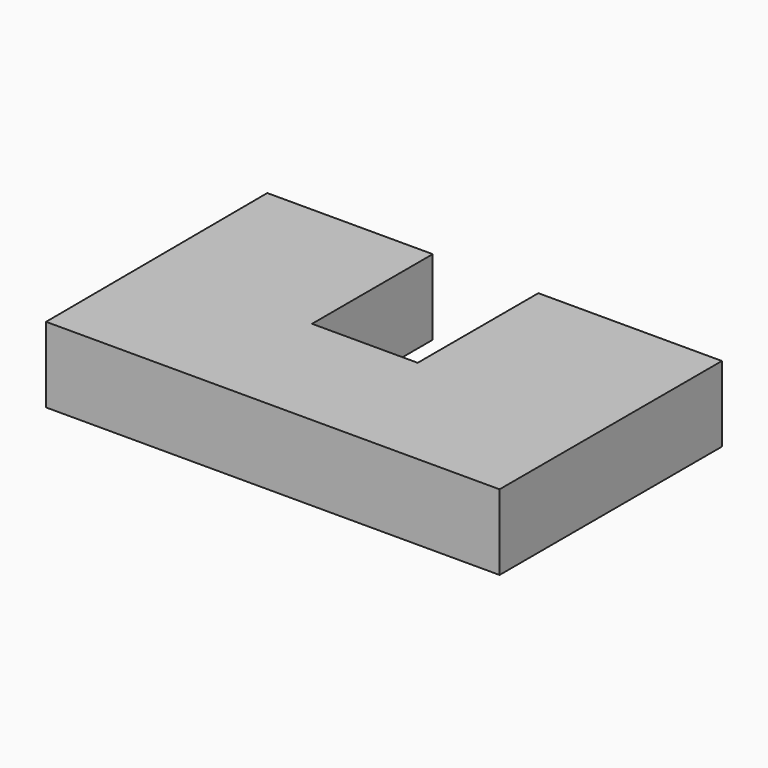
from build123d import *

# Parameters (mm, degrees)
F1_DEPTH = 25
F2_W     = 35.0194228813
F2_H     = 50
F3_DEPTH = 40.3


# Not quite as in the source:
# - the program builds the solid bodies; features that only make, move or delete a surface that nothing else refers to are left out


with BuildPart() as f1:
    # F0 (on Top) → F1 (new body)
    with BuildSketch(Plane.XY):
        Polygon((75.4525884986, 36.6594865918), (-75.2586200833, 36.6594865918), (-74.8706907034, -55.47413975), (75.4525884986, -55.47413975), align=None)
    extrude(amount=F1_DEPTH)

    # F2 (on face) → F3 (cut)
    with BuildSketch(Plane.XY.offset(25)):
        with Locations((-2.906773705, 11.6594865918)):
            Rectangle(F2_W, F2_H)
    extrude(amount=-F3_DEPTH, mode=Mode.SUBTRACT)


solid = f1.part
